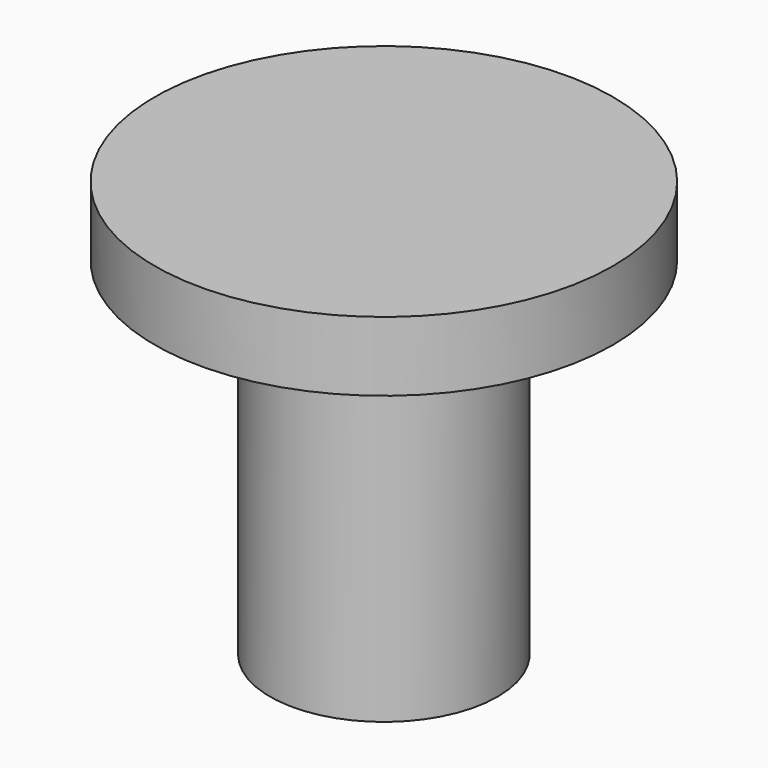
from build123d import *

# Parameters (mm, degrees)
F2_R     = 16.5
F3_DEPTH = 5
F4_R     = 8.2
F4_R_2   = 7.7
F5_DEPTH = 25


# Not quite as in the source:
# - the program builds the solid bodies; features that only make, move or delete a surface that nothing else refers to are left out


with BuildPart() as f3:
    # F2 (on Top) → F3 (new body)
    with BuildSketch(Plane.XY):
        with Locations((-45.8642121462, 17.7900076957)):
            Circle(F2_R)
    extrude(amount=F3_DEPTH)

    # F4 (on Top) → F5 (join)
    with BuildSketch(Plane.XY):
        with Locations((-45.8642121462, 17.7900076957)):
            Circle(F4_R)
        with Locations((-45.8642121462, 17.7900076957)):
            Circle(F4_R_2, mode=Mode.SUBTRACT)
    extrude(amount=-F5_DEPTH)


solid = f3.part
